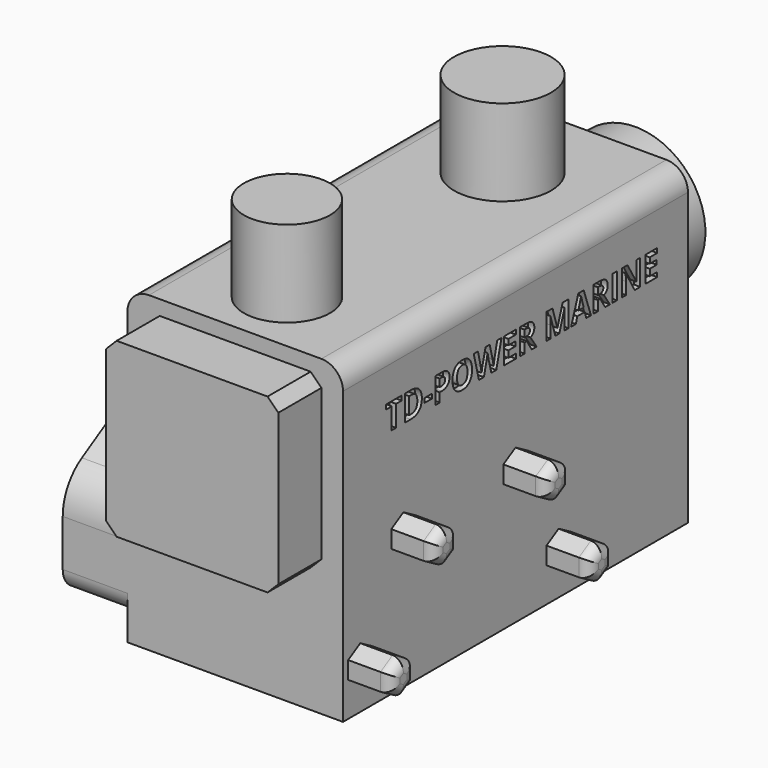
from build123d import *

# Parameters (mm, degrees)
F0_W         = 200
F0_H         = 145
F1_DEPTH     = 100
F2_R         = 20
F2_R_2       = 22.5
F3_DEPTH     = 40
F4_W         = 80
F4_H         = 80
F4_H_2       = 50
F5_DEPTH     = 7
F6_R         = 32.5
F7_DEPTH     = 25
F8_TEXT_SIZE = 16.6666666667
F9_DEPTH     = 3
F11_DEPTH    = 20
F12_R        = 5
F13_W        = 80
F13_H        = 80
F14_DEPTH    = 25
F15_SIZE     = 5
F16_R        = 10
F17_R        = 15
F18_DEPTH    = 30


# Not quite as in the source:
# - Text() gives the source's letters only with a copy of the font that has no kerning and outlines rounded to 1/6400 em; it was checked with that copy


with BuildPart() as f1:
    # F0 (on Right) → F1 (new body)
    with BuildSketch(Plane.YZ):
        Rectangle(F0_W, F0_H)
    extrude(amount=F1_DEPTH)

    # F2 (on face) → F3 (join)
    with BuildSketch(Plane.XY.offset(72.5)):
        with Locations((50, -70)):
            Circle(F2_R)
        with Locations((50, 55)):
            Circle(F2_R_2)
    extrude(amount=F3_DEPTH)

    # F4 (on face) → F5 (join)
    with BuildSketch(Plane(origin=(0, 100, 0), x_dir=(-1, 0, 0), z_dir=(0, 1, 0))):
        with Locations((-50, 27.4677090347)):
            Rectangle(F4_W, F4_H)
        with Locations((-50, -41.5475107729)):
            Rectangle(F4_W, F4_H_2)
    extrude(amount=F5_DEPTH)

    # F6 (on face) → F7 (join)
    with BuildSketch(Plane(origin=(0, 107, 0), x_dir=(-1, 0, 0), z_dir=(0, 1, 0))):
        with Locations((-50, 27.4677090347)):
            Circle(F6_R)
    extrude(amount=F7_DEPTH)

    # F8 (on face) → F9 (cut)
    with BuildSketch(Plane.YZ.offset(100)):
        with Locations((-75.3048277339, 35.0813497917)):
            Text('TD-POWER MARINE', F8_TEXT_SIZE, font='Open Sans', font_style=FontStyle.BOLD, text_align=(TextAlign.LEFT, TextAlign.BOTTOM))
    extrude(amount=-F9_DEPTH, mode=Mode.SUBTRACT)

    # F10 (on face) → F11 (join)
    with BuildSketch(Plane.YZ.offset(100)):
        Polygon((-83, -56.5414518843), (-83, -48.4585481157), (-90, -44.4170962313), (-97, -48.4585481157), (-97, -56.5414518843), (-90, -60.5829037687), align=None)
        Polygon((32, -56.5414518843), (32, -48.4585481157), (25, -44.4170962313), (18, -48.4585481157), (18, -56.5414518843), (25, -60.5829037687), align=None)
        Polygon((-64.9999996883, -17.2816335794), (-57.9999998441, -13.2401814252), (-58.0000001559, -5.1572776565), (-65.0000003117, -1.1158260421), (-72.0000001559, -5.1572781964), (-71.9999998441, -13.240181965), align=None)
        Polygon((7, -13.2401816951), (7, -5.1572779265), (0, -1.1158260421), (-7, -5.1572779265), (-7, -13.2401816951), (0, -17.2816335794), align=None)
    extrude(amount=F11_DEPTH)

    # F12
    f12_edges = [f1.edges().sort_by_distance(p)[0] for p in [
        (120, -86.5, -58.562178),
        (120, -83, -52.5),
        (120, -86.5, -46.437822),
        (120, -93.5, -46.437822),
        (120, -97, -52.5),
        (120, -93.5, -58.562178),
        (120, -61.5, -15.260908),
        (120, -58, -9.19873),
        (120, -61.5, -3.136552),
        (120, -68.5, -3.136552),
        (120, -72, -9.19873),
        (120, -68.5, -15.260908),
        (120, 7, -9.19873),
        (120, 3.5, -3.136552),
        (120, -3.5, -3.136552),
        (120, -7, -9.19873),
        (120, -3.5, -15.260908),
        (120, 3.5, -15.260908),
        (120, 32, -52.5),
        (120, 28.5, -46.437822),
        (120, 21.5, -46.437822),
        (120, 18, -52.5),
        (120, 21.5, -58.562178),
        (120, 28.5, -58.562178),
    ]]
    fillet(f12_edges, radius=F12_R)

    # F13 (on face) → F14 (join)
    with BuildSketch(Plane.XZ.offset(100)):
        with Locations((50, 25.6515145302)):
            Rectangle(F13_W, F13_H)
    extrude(amount=F14_DEPTH)

    # F15
    f15_edges = [f1.edges().sort_by_distance(p)[0] for p in [
        (90, -112.5, 65.651515),
        (90, -112.5, -14.348485),
        (10, -112.5, -14.348485),
        (10, -112.5, 65.651515),
        (90, 103.5, 67.467709),
        (10, 103.5, 67.467709),
        (90, 103.5, -12.532291),
        (10, 103.5, -12.532291),
    ]]
    chamfer(f15_edges, length=F15_SIZE)

    # F16
    f16_edges = [f1.edges().sort_by_distance(p)[0] for p in [
        (100, 0, 72.5),
        (0, 0, 72.5),
    ]]
    fillet(f16_edges, radius=F16_R)

    # F17 (on face) → F18 (join)
    with BuildSketch(Plane(origin=(0, 0, 0), x_dir=(0, -1, 0), z_dir=(-1, 0, 0))):
        with BuildLine():
            Line((54.8880097821, -10.1081523472), (55.0003260636, -30.9704960567))
            ThreePointArc((55.0003260636, -30.9704960567), (58.0447819074, -42.1517756645), (66.25, -50.3349364905))
            Line((66.25, -50.3349364905), (85, -61.1602540378))
            ThreePointArc((85, -61.1602540378), (95, -61.1602540378), (100, -52.5))
            Line((100, -52.5), (100, -30.8493649054))
            ThreePointArc((100, -30.8493649054), (97.025052192, -19.668026126), (88.8869033868, -11.4434783949))
            Line((88.8869033868, -11.4434783949), (70.106114359, -0.423367045))
            ThreePointArc((70.106114359, -0.423367045), (59.5489941418, -0.6333383631), (54.8880097821, -10.1081523472))
        make_face()
        with Locations((77.5, -30.8493649054)):
            Circle(F17_R, mode=Mode.SUBTRACT)
        with BuildLine():
            Line((9.9394439915, -34.1496524947), (9.9999705197, -9.2230116023))
            ThreePointArc((9.9999705197, -9.2230116023), (4.7300920546, -0.3881549626), (-5.5454683331, -0.8772046521))
            Line((-5.5454683331, -0.8772046521), (-23.8158484859, -13.0525946963))
            ThreePointArc((-23.8158484859, -13.0525946963), (-31.5799618401, -20.5750238499), (-34.9394439915, -30.8503475053))
            Line((-34.9394439915, -30.8503475053), (-34.9999608311, -52.4720111257))
            ThreePointArc((-34.9999608311, -52.4720111257), (-30.2999894, -60.9799830401), (-20.5928361533, -61.4764640493))
            Line((-20.5928361533, -61.4764640493), (-1.1841515141, -51.9474053037))
            ThreePointArc((-1.1841515141, -51.9474053037), (6.5799618401, -44.4249761501), (9.9394439915, -34.1496524947))
        make_face()
        with Locations((-12.5, -30.8493649054)):
            Circle(F17_R, mode=Mode.SUBTRACT)
    extrude(amount=F18_DEPTH)


solid = f1.part
